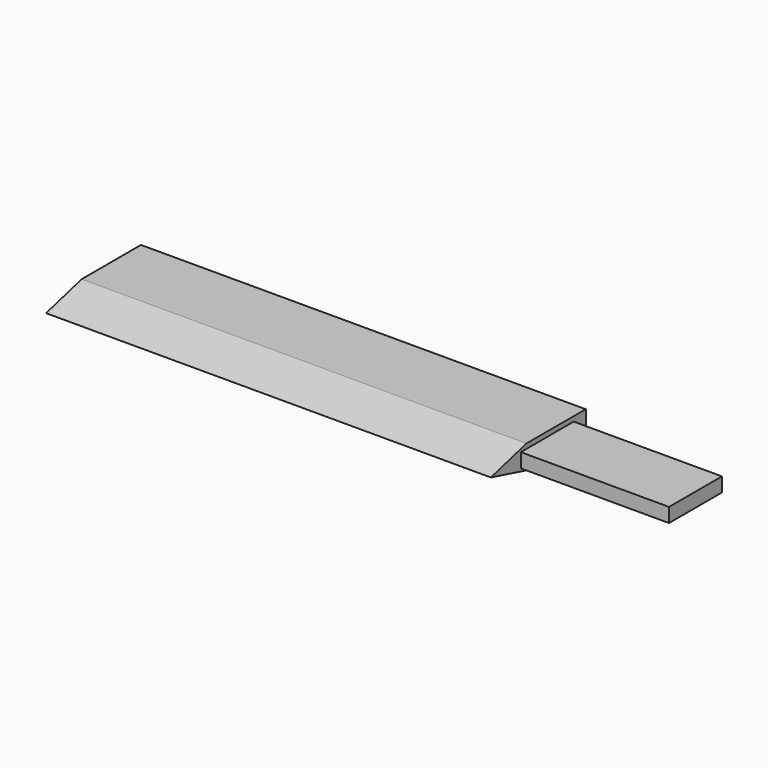
from build123d import *

# Parameters (mm, degrees)
F0_W     = 150
F0_H     = 40
F1_DEPTH = 8
F2_SIZE2 = 14.99999
F2_SIZE  = 3.99999
F4_DEPTH = 70
F6_DEPTH = 50


# Not quite as in the source:
# - a fillet or chamfer is up to 0.001 mm smaller than in the source, because OpenCascade refuses the exact size


with BuildPart() as f1:
    # F0 (on Top) → F1 (new body)
    with BuildSketch(Plane.XY):
        with Locations((-75, 20)):
            Rectangle(F0_W, F0_H)
    extrude(amount=F1_DEPTH)

    # F2 (size 4 and 15 in the source; OpenCascade refuses exactly that, so slightly less here)
    f2_edges = [f1.edges().sort_by_distance(p)[0] for p in [
        (-75, 0, 8),
        (-75, 0, 0),
    ]]
    f2_side = f1.faces().sort_by_distance((-75, 0, 4))[0]
    chamfer(f2_edges, length=F2_SIZE, length2=F2_SIZE2, reference=f2_side)

    # F3 (on face) → F4 (cut)
    with BuildSketch(Plane(origin=(-150, 0, 0), x_dir=(0, -1, 0), z_dir=(-1, 0, 0))):
        Polygon((-12.5, 1.5), (-12.5, 4), (-12.5, 6.5), (-35, 6.5), (-35, 1.5), align=None)
    extrude(amount=-F4_DEPTH, mode=Mode.SUBTRACT)

    # F5 (on face) → F6 (join)
    with BuildSketch(Plane.YZ):
        Polygon((12.6, 6.4), (12.6, 4), (12.6, 1.6), (34.9, 1.6), (34.9, 6.4), align=None)
    extrude(amount=F6_DEPTH)


solid = f1.part
